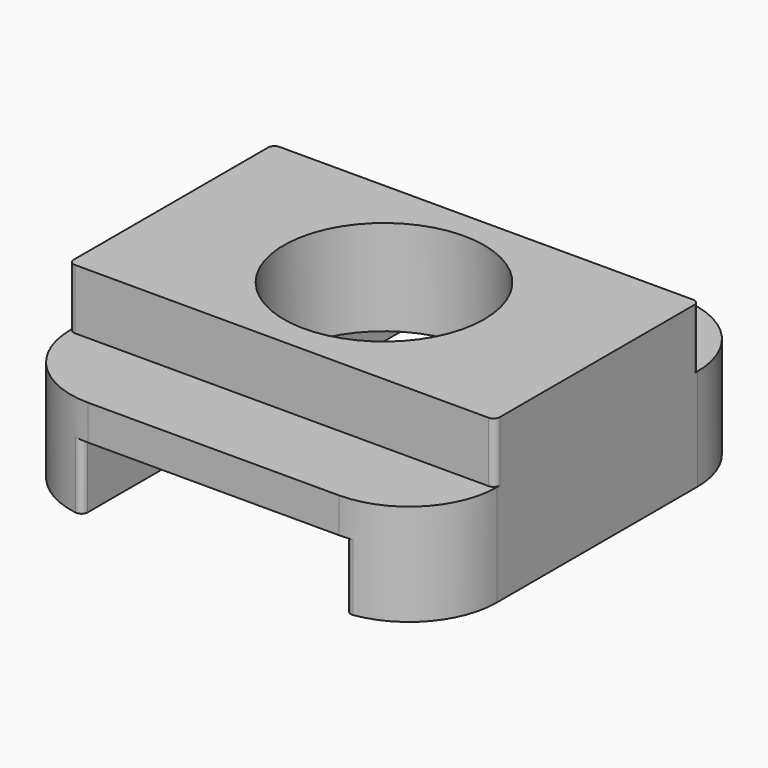
from build123d import *

# Parameters (mm, degrees)
F0_W        = 34
F0_H        = 34
F1_DEPTH    = 12.9
F2_W        = 21
F2_H        = 5.3
F3_DEPTH    = 34.001
F4_W        = 6.8
F4_H        = 4.8
F5_DEPTH    = 34.001
F6_R        = 8
F7_DEPTH    = 12.901
F8_R        = 7
F9_T1_DEPTH = 6.0500204163
F9_T3_DEPTH = 6.751561158


# Not quite as in the source:
# - a fillet or chamfer that OpenCascade refuses, or shapes differently, is made with other operations: its cross-section is extruded or revolved along the edge and cut away or added


with BuildPart() as f1:
    # F0 (on Top) → F1 (new body)
    with BuildSketch(Plane.XY):
        Rectangle(F0_W, F0_H)
    extrude(amount=F1_DEPTH)

    # F2 (on face) → F3 (cut, through all)
    with BuildSketch(Plane.XZ.offset(17)):
        with Locations((0, 2.65)):
            Rectangle(F2_W, F2_H)
    extrude(amount=-F3_DEPTH, mode=Mode.SUBTRACT)

    # F4 (on face) → F5 (cut, through all)
    with BuildSketch(Plane.YZ.offset(17)):
        with Locations((-13.6, 10.5)):
            Rectangle(F4_W, F4_H)
        with Locations((13.6, 10.5)):
            Rectangle(F4_W, F4_H)
    extrude(amount=-F5_DEPTH, mode=Mode.SUBTRACT)

    # F6 (on face) → F7 (cut, through all)
    with BuildSketch(Plane.XY.offset(12.9)):
        Circle(F6_R)
    extrude(amount=-F7_DEPTH, mode=Mode.SUBTRACT)

    # F8
    f8_edges = [f1.edges().sort_by_distance(p)[0] for p in [
        (17, -17, 4.05),
        (17, 17, 4.05),
        (-17, -17, 4.05),
        (-17, 17, 4.05),
    ]]
    fillet(f8_edges, radius=F8_R)

    # F9: fillet of radius 0.5 on 8 edges, made by hand

    # F9_s2 → F9_t1 (cut)
    with BuildSketch(Plane.XY.offset(8.1)):
        with BuildLine():
            ThreePointArc((17, -9.7), (16.8535533906, -10.0535533906), (16.5, -10.2))
            Line((16.5, -10.2), (16.5, -10.25))
            Line((16.5, -10.25), (16.9971422738, -10.25))
            Line((16.9971422738, -10.25), (17.0471218615, -10.2014285714))
            ThreePointArc((17.0471218615, -10.2014285714), (17.05, -10), (17.05, -9.7))
            Line((17.05, -9.7), (17, -9.7))
        make_face()
        with BuildLine():
            ThreePointArc((17, 9.7), (16.8535533906, 10.0535533906), (16.5, 10.2))
            Line((16.5, 10.2), (16.5, 10.25))
            Line((16.5, 10.25), (16.9971422738, 10.25))
            Line((16.9971422738, 10.25), (17.0471218615, 10.2014285714))
            ThreePointArc((17.0471218615, 10.2014285714), (17.05, 10), (17.05, 9.7))
            Line((17.05, 9.7), (17, 9.7))
        make_face()
        with BuildLine():
            ThreePointArc((-17, 9.7), (-16.8535533906, 10.0535533906), (-16.5, 10.2))
            Line((-16.5, 10.2), (-16.5, 10.25))
            Line((-16.5, 10.25), (-16.9971422738, 10.25))
            Line((-16.9971422738, 10.25), (-17.0471218615, 10.2014285714))
            ThreePointArc((-17.0471218615, 10.2014285714), (-17.05, 10), (-17.05, 9.7))
            Line((-17.05, 9.7), (-17, 9.7))
        make_face()
        with BuildLine():
            ThreePointArc((-17, -9.7), (-16.8535533906, -10.0535533906), (-16.5, -10.2))
            Line((-16.5, -10.2), (-16.5, -10.25))
            Line((-16.5, -10.25), (-16.9971422738, -10.25))
            Line((-16.9971422738, -10.25), (-17.0471218615, -10.2014285714))
            ThreePointArc((-17.0471218615, -10.2014285714), (-17.05, -10), (-17.05, -9.7))
            Line((-17.05, -9.7), (-17, -9.7))
        make_face()
    extrude(amount=F9_T1_DEPTH, mode=Mode.SUBTRACT)

    # F9_s4 → F9_t3 (cut)
    with BuildSketch(Plane.XY.offset(-1.451561158)):
        with BuildLine():
            ThreePointArc((11.0769230769, -16.9166636962), (10.6747781822, -16.802393552), (10.5, -16.4226162893))
            Line((10.5, -16.4226162893), (10.5, -16.9821200219))
            ThreePointArc((10.5, -16.9821200219), (10.789140501, -16.9553761415), (11.0769230769, -16.9166636962))
        make_face()
        with BuildLine():
            ThreePointArc((-11.0769230769, -16.9166636962), (-10.6747781822, -16.802393552), (-10.5, -16.4226162893))
            Line((-10.5, -16.4226162893), (-10.5, -16.9821200219))
            ThreePointArc((-10.5, -16.9821200219), (-10.789140501, -16.9553761415), (-11.0769230769, -16.9166636962))
        make_face()
        with BuildLine():
            ThreePointArc((-11.0769230769, 16.9166636962), (-10.6747781822, 16.802393552), (-10.5, 16.4226162893))
            Line((-10.5, 16.4226162893), (-10.5, 16.9821200219))
            ThreePointArc((-10.5, 16.9821200219), (-10.789140501, 16.9553761415), (-11.0769230769, 16.9166636962))
        make_face()
        with BuildLine():
            ThreePointArc((11.0769230769, 16.9166636962), (10.6747781822, 16.802393552), (10.5, 16.4226162893))
            Line((10.5, 16.4226162893), (10.5, 16.9821200219))
            ThreePointArc((10.5, 16.9821200219), (10.789140501, 16.9553761415), (11.0769230769, 16.9166636962))
        make_face()
    extrude(amount=F9_T3_DEPTH, mode=Mode.SUBTRACT)


solid = f1.part
